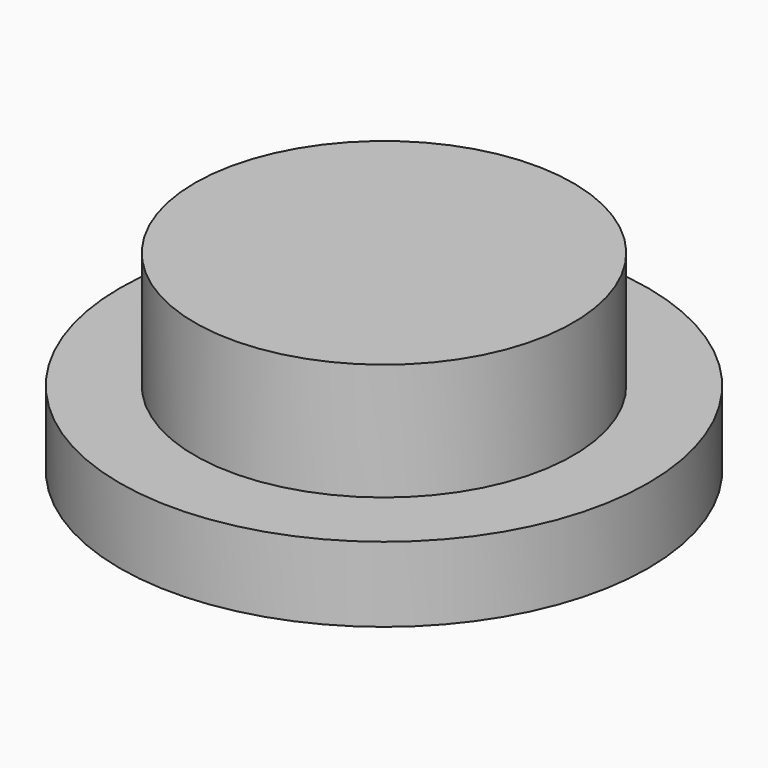
from build123d import *

# Parameters (mm, degrees)
F2_TEXT_SIZE = 12.9117356395
F3_DEPTH     = 0.508


# Not quite as in the source:
# - Text() gives the source's letters only with a copy of the font that has no kerning and outlines rounded to 1/6400 em; it was checked with that copy


with BuildPart() as f1:
    # F0 (on Front) → F1 (revolve)
    with BuildSketch(Plane.XZ):
        Polygon((-8.9535, 0), (0, 0), (0, 6.5024), (-6.4135, 6.5024), (-6.4135, 2.54), (-8.9535, 2.54), align=None)
    revolve(axis=Axis((0, 0, 4.0118594139), (0, 0, 1)))

    # F2 (on face) → F3 (cut)
    with BuildSketch(Plane(origin=(0, 0, 0), x_dir=(1, 0, 0), z_dir=(0, 0, -1))):
        with Locations((-7.1932489723, -4.6482248302)):
            Text('TF', F2_TEXT_SIZE, font='Open Sans', text_align=(TextAlign.LEFT, TextAlign.BOTTOM))
    extrude(amount=-F3_DEPTH, mode=Mode.SUBTRACT)


solid = f1.part
